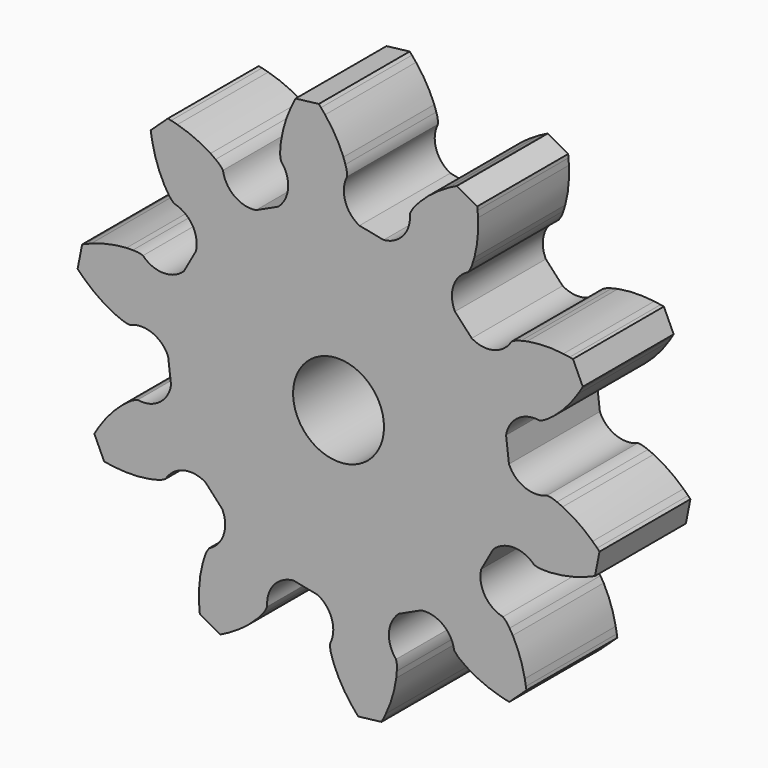
from build123d import *

# Parameters (mm, degrees)
F0_R     = 2
F1_DEPTH = 5


# Not quite as in the source:
# - ends of sketch curves that miss each other by under 0.0002 mm in the source are joined


with BuildPart() as f1:
    # F0 (on Front) → F1 (new body)
    with BuildSketch(Plane.XZ):
        with BuildLine():
            ThreePointArc((3.1397715417, 8.6264479588), (2.8484773823, 7.694719731), (1.9836699588, 7.2418644583))
            Line((1.9836699588, 7.2418644583), (0.918632, 7.452224))
            ThreePointArc((0.918632, 7.452224), (0.2909434317, 8.1998690692), (0.3757643758, 9.1723788045))
            ThreePointArc((0.3757643758, 9.1723788045), (0.3597750699, 9.3990684228), (0.299837375, 9.6182731434))
            Line((0.299837375, 9.6182731434), (0.214416, 9.878691))
            ThreePointArc((0.214416, 9.878691), (-0.1356548668, 10.5984980157), (-0.5914550473, 11.2564619615))
            Line((-0.5914550473, 11.2564619615), (-0.771673, 11.473606))
            Line((-0.771673, 11.473606), (-0.869145, 11.583845))
            Line((-0.869145, 11.583845), (-1.889897, 11.461641))
            Line((-1.889897, 11.461641), (-1.958592, 11.331507))
            Line((-1.958592, 11.331507), (-2.082456, 11.077956))
            ThreePointArc((-2.082456, 11.077956), (-2.3700557848, 10.3309889247), (-2.540316378, 9.5488880524))
            Line((-2.540316378, 9.5488880524), (-2.56185, 9.275668))
            ThreePointArc((-2.56185, 9.275668), (-2.5683473923, 9.0485086782), (-2.5303705918, 8.8244531113))
            ThreePointArc((-2.5303705918, 8.8244531113), (-2.2183773042, 7.8994524474), (-2.6518400095, 7.0247640109))
            Line((-2.6518400095, 7.0247640109), (-3.637119, 6.568934))
            ThreePointArc((-3.637119, 6.568934), (-4.5843861873, 6.8048471816), (-5.0873915713, 7.6414810642))
            ThreePointArc((-5.0873915713, 7.6414810642), (-5.2335689379, 7.8154766592), (-5.4109047291, 7.9575864159))
            Line((-5.4109047291, 7.9575864159), (-5.633082, 8.118061))
            ThreePointArc((-5.633082, 8.118061), (-6.3393864036, 8.4946269969), (-7.0948779027, 8.7590183656))
            Line((-7.0948779027, 8.7590183656), (-7.368313, 8.828765))
            Line((-7.368313, 8.828765), (-7.511967, 8.860658))
            Line((-7.511967, 8.860658), (-8.265942, 8.161806))
            Line((-8.265942, 8.161806), (-8.245026, 8.016152))
            Line((-8.245026, 8.016152), (-8.196201, 7.738217))
            ThreePointArc((-8.196201, 7.738217), (-7.9898196328, 6.964862558), (-7.6678559525, 6.2320530254))
            Line((-7.6678559525, 6.2320530254), (-7.524681, 5.998354))
            ThreePointArc((-7.524681, 5.998354), (-7.3964178738, 5.810760264), (-7.2339973764, 5.6518175311))
            ThreePointArc((-7.2339973764, 5.6518175311), (-6.4378867329, 5.0868607506), (-6.2744360854, 4.1244400195))
            Line((-6.2744360854, 4.1244400195), (-6.803613, 3.176535))
            ThreePointArc((-6.803613, 3.176535), (-7.7086336789, 2.8106016294), (-8.607334508, 3.1917934837))
            ThreePointArc((-8.607334508, 3.1917934837), (-8.8278689728, 3.2466380541), (-9.0548669954, 3.2573719089))
            Line((-9.0548669954, 3.2573719089), (-9.328934, 3.256607))
            ThreePointArc((-9.328934, 3.256607), (-10.1216881787, 3.1460992273), (-10.888299197, 2.9159295105))
            Line((-10.888299197, 2.9159295105), (-11.150508, 2.811637))
            Line((-11.150508, 2.811637), (-11.285472, 2.752999))
            Line((-11.285472, 2.752999), (-11.484678, 1.744441))
            Line((-11.484678, 1.744441), (-11.382143, 1.638897))
            Line((-11.382143, 1.638897), (-11.179276, 1.442742))
            ThreePointArc((-11.179276, 1.442742), (-10.5577420476, 0.938395095), (-9.8665329482, 0.5347851067))
            Line((-9.8665329482, 0.5347851067), (-9.613338, 0.429873))
            ThreePointArc((-9.613338, 0.429873), (-9.3993074084, 0.3534985414), (-9.1744820206, 0.3203795712))
            ThreePointArc((-9.1744820206, 0.3203795712), (-8.1983406498, 0.3312616644), (-7.5004096996, -0.351279299))
            Line((-7.5004096996, -0.351279299), (-7.37136, -1.429192))
            ThreePointArc((-7.37136, -1.429192), (-7.8884451663, -2.2571976007), (-8.8395680123, -2.4770500734))
            ThreePointArc((-8.8395680123, -2.4770500734), (-9.0502220136, -2.5623049352), (-9.2401760461, -2.6870469429))
            Line((-9.2401760461, -2.6870469429), (-9.461451, -2.848761))
            ThreePointArc((-9.461451, -2.848761), (-10.0378498301, -3.4041288223), (-10.5227607427, -4.0409425195))
            Line((-10.5227607427, -4.0409425195), (-10.67359, -4.279445))
            Line((-10.67359, -4.279445), (-10.748312, -4.40621))
            Line((-10.748312, -4.40621), (-10.316657, -5.33924))
            Line((-10.316657, -5.33924), (-10.171665, -5.36436))
            Line((-10.171665, -5.36436), (-9.892247, -5.403809))
            ThreePointArc((-9.892247, -5.403809), (-9.0929671722, -5.446510229), (-8.2965319488, -5.366755287))
            Line((-8.2965319488, -5.366755287), (-8.030028, -5.302804))
            ThreePointArc((-8.030028, -5.302804), (-7.8119805721, -5.238787582), (-7.6106266058, -5.1334326012))
            ThreePointArc((-7.6106266058, -5.1334326012), (-6.8273082533, -4.5508675638), (-5.8614831335, -4.6928212233))
            Line((-5.8614831335, -4.6928212233), (-5.123497, -5.489017))
            ThreePointArc((-5.123497, -5.489017), (-5.0551391941, -6.4628231896), (-5.6953873364, -7.1997433257))
            ThreePointArc((-5.6953873364, -7.1997433257), (-5.8156976419, -7.392534822), (-5.8960523452, -7.605105907))
            Line((-5.8960523452, -7.605105907), (-5.980015, -7.865997))
            ThreePointArc((-5.980015, -7.865997), (-6.1198933621, -8.6540995562), (-6.1378847427, -9.4543160402))
            Line((-6.1378847427, -9.4543160402), (-6.119721, -9.735921))
            Line((-6.119721, -9.735921), (-6.105661, -9.882399))
            Line((-6.105661, -9.882399), (-5.208024, -10.383515))
            Line((-5.208024, -10.383515), (-5.075958, -10.318614))
            Line((-5.075958, -10.318614), (-4.826716, -10.18629))
            ThreePointArc((-4.826716, -10.18629), (-4.1549863609, -9.751031687), (-3.5575354172, -9.2183755607))
            Line((-3.5575354172, -9.2183755607), (-3.379521, -9.00999))
            ThreePointArc((-3.379521, -9.00999), (-3.2407424242, -8.8300347429), (-3.1397695271, -8.6264471792))
            ThreePointArc((-3.1397695271, -8.6264471792), (-2.8484743823, -7.694719731), (-1.9836669588, -7.2418644583))
            Line((-1.9836669588, -7.2418644583), (-0.918631, -7.452225))
            ThreePointArc((-0.918631, -7.452225), (-0.2909405652, -8.1998706462), (-0.3757613758, -9.1723808045))
            ThreePointArc((-0.3757613758, -9.1723808045), (-0.3597760676, -9.3990684365), (-0.299838375, -9.6182731434))
            Line((-0.299838375, -9.6182731434), (-0.214416, -9.878689))
            ThreePointArc((-0.214416, -9.878689), (0.135655026, -10.5984962879), (0.5914554451, -11.256460451))
            Line((0.5914554451, -11.256460451), (0.771674, -11.473608))
            Line((0.771674, -11.473608), (0.869145, -11.583847))
            Line((0.869145, -11.583847), (1.8899, -11.461641))
            Line((1.8899, -11.461641), (1.958593, -11.331507))
            Line((1.958593, -11.331507), (2.082459, -11.077955))
            ThreePointArc((2.082459, -11.077955), (2.3700558045, -10.3309888589), (2.5403163969, -9.5488879164))
            Line((2.5403163969, -9.5488879164), (2.561849, -9.275668))
            ThreePointArc((2.561849, -9.275668), (2.5683503831, -9.048508547), (2.5303735226, -8.8244528575))
            ThreePointArc((2.5303735226, -8.8244528575), (2.2183762789, -7.8994508231), (2.6518384423, -7.0247625063))
            Line((2.6518384423, -7.0247625063), (3.637117, -6.568934))
            ThreePointArc((3.637117, -6.568934), (4.5843865849, -6.8048454757), (5.0873915713, -7.6414790642))
            ThreePointArc((5.0873915713, -7.6414790642), (5.2335709379, -7.8154766592), (5.4109067291, -7.9575864159))
            Line((5.4109067291, -7.9575864159), (5.633082, -8.118059))
            ThreePointArc((5.633082, -8.118059), (6.3393874036, -8.4946269969), (7.0948789027, -8.7590183656))
            Line((7.0948789027, -8.7590183656), (7.368313, -8.828765))
            Line((7.368313, -8.828765), (7.511968, -8.860658))
            Line((7.511968, -8.860658), (8.265941, -8.161808))
            Line((8.265941, -8.161808), (8.245029, -8.016151))
            Line((8.245029, -8.016151), (8.196202, -7.738217))
            ThreePointArc((8.196202, -7.738217), (7.9898196328, -6.964862558), (7.6678559525, -6.2320530254))
            Line((7.6678559525, -6.2320530254), (7.524682, -5.998354))
            ThreePointArc((7.524682, -5.998354), (7.3964187194, -5.8107600798), (7.2339983764, -5.6518175311))
            ThreePointArc((7.2339983764, -5.6518175311), (6.4378855328, -5.0868604321), (6.2744350358, -4.1244402365))
            Line((6.2744350358, -4.1244402365), (6.803614, -3.176535))
            ThreePointArc((6.803614, -3.176535), (7.7086359718, -2.8106016234), (8.6073370165, -3.1917929838))
            ThreePointArc((8.6073370165, -3.1917929838), (8.8278694641, -3.2466381261), (9.0548670463, -3.2573719063))
            Line((9.0548670463, -3.2573719063), (9.328933, -3.256605))
            ThreePointArc((9.328933, -3.256605), (10.1216871787, -3.1461012273), (10.888298197, -2.9159315105))
            Line((10.888298197, -2.9159315105), (11.150511, -2.811635))
            Line((11.150511, -2.811635), (11.285475, -2.753))
            Line((11.285475, -2.753), (11.484676, -1.744443))
            Line((11.484676, -1.744443), (11.382143, -1.638897))
            Line((11.382143, -1.638897), (11.179276, -1.442742))
            ThreePointArc((11.179276, -1.442742), (10.5577424175, -0.9383933509), (9.8665337575, -0.5347834996))
            Line((9.8665337575, -0.5347834996), (9.613339, -0.429875))
            ThreePointArc((9.613339, -0.429875), (9.3993079697, -0.353498432), (9.1744830206, -0.3203795712))
            ThreePointArc((9.1744830206, -0.3203795712), (8.1983388321, -0.3312617375), (7.500407854, 0.3512789376))
            Line((7.500407854, 0.3512789376), (7.371361, 1.429192))
            ThreePointArc((7.371361, 1.429192), (7.8884460322, 2.257197505), (8.8395688497, 2.4770501006))
            ThreePointArc((8.8395688497, 2.4770501006), (9.0502222442, 2.5623065319), (9.2401764408, 2.6870484541))
            Line((9.2401764408, 2.6870484541), (9.46145, 2.848759))
            ThreePointArc((9.46145, 2.848759), (10.037850267, 3.4041313131), (10.5227610378, 4.0409449756))
            Line((10.5227610378, 4.0409449756), (10.67359, 4.279443))
            Line((10.67359, 4.279443), (10.748313, 4.406212))
            Line((10.748313, 4.406212), (10.316657, 5.339242))
            Line((10.316657, 5.339242), (10.171666, 5.36436))
            Line((10.171666, 5.36436), (9.892248, 5.403811))
            ThreePointArc((9.892248, 5.403811), (9.0929676801, 5.4465102176), (8.2965319796, 5.3667551142))
            Line((8.2965319796, 5.3667551142), (8.030031, 5.302802))
            ThreePointArc((8.030031, 5.302802), (7.8119811844, 5.2387874254), (7.6106269064, 5.1334321427))
            ThreePointArc((7.6106269064, 5.1334321427), (6.8273086695, 4.5508656686), (5.8614831335, 4.6928192233))
            Line((5.8614831335, 4.6928192233), (5.123498, 5.489019))
            ThreePointArc((5.123498, 5.489019), (5.0551411941, 6.4628251896), (5.6953893364, 7.1997453257))
            ThreePointArc((5.6953893364, 7.1997453257), (5.8156986419, 7.392536822), (5.8960533452, 7.605107907))
            Line((5.8960533452, 7.605107907), (5.980014, 7.865997))
            ThreePointArc((5.980014, 7.865997), (6.1198932745, 8.6540996749), (6.1378847997, 9.4543159891))
            Line((6.1378847997, 9.4543159891), (6.119721, 9.735921))
            Line((6.119721, 9.735921), (6.105663, 9.882397))
            Line((6.105663, 9.882397), (5.208024, 10.383517))
            Line((5.208024, 10.383517), (5.075961, 10.318613))
            Line((5.075961, 10.318613), (4.826717, 10.186292))
            ThreePointArc((4.826717, 10.186292), (4.154986926, 9.7510293554), (3.5575359365, 9.2183730611))
            Line((3.5575359365, 9.2183730611), (3.379519, 9.009988))
            ThreePointArc((3.379519, 9.009988), (3.2407432425, 8.8300344523), (3.1397715417, 8.6264479588))
        make_face()
        with Locations((-1e-06, 0)):
            Circle(F0_R, mode=Mode.SUBTRACT)
    extrude(amount=F1_DEPTH)


solid = f1.part
